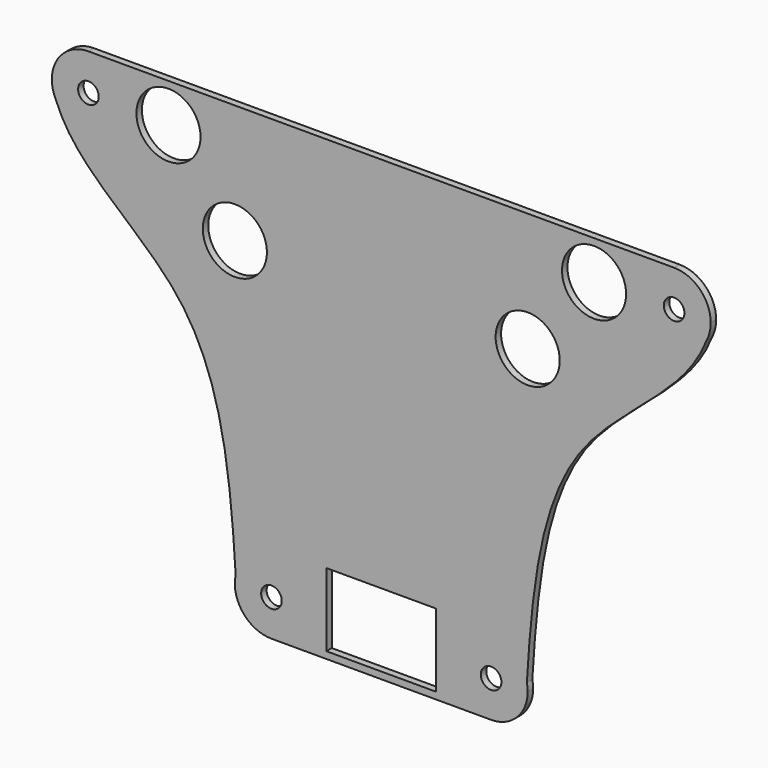
from build123d import *

# Parameters (mm, degrees)
F0_R     = 7.1501
F0_R_2   = 22.2504
F1_DEPTH = 4.7498


with BuildPart() as f1:
    # F0 (on Front) → F1 (new body)
    with BuildSketch(Plane.XZ):
        with BuildLine():
            ThreePointArc((-225.6573369788, 94.4161567678), (-197.0867504248, 81.6298943923), (-177.8, 106.2832548048))
            ThreePointArc((-177.8, 106.2832548048), (-185.2394877579, 124.2437670469), (-203.2, 131.6832548048))
            ThreePointArc((-203.2, 131.6832548048), (-224.9552785565, 119.3930929018), (-225.6573369788, 94.4161567678))
        make_face()
        with Locations((-203.2, 106.2832548048)):
            Circle(F0_R, mode=Mode.SUBTRACT)
        with BuildLine():
            ThreePointArc((-203.2, 131.6832548048), (-185.2394877579, 124.2437670469), (-177.8, 106.2832548048))
            ThreePointArc((-177.8, 106.2832548048), (-197.0867504248, 81.6298943923), (-225.6573369788, 94.4161567678))
            add(Edge.make_bspline(
                [(-225.6573369788, 94.4161567678), (-210.8833649868, 55.9874046479), (-115.4710726931, 10.7964254469), (-104.8309285082, -94.2151341667), (-101.0213270695, -155.0258526432)],
                knots=[0, 0, 0, 0, 0.4720003547, 1, 1, 1, 1], degree=3))
            ThreePointArc((-101.0213270695, -155.0258526432), (-73.4890691235, -135.1618277773), (-50.8, -160.4167451952))
            ThreePointArc((-50.8, -160.4167451952), (-58.2394877579, -178.3772574373), (-76.2, -185.8167451952))
            Line((-76.2, -185.8167451952), (76.2, -185.8167451952))
            ThreePointArc((76.2, -185.8167451952), (56.4251590294, -144.4757394368), (101.0213270695, -155.0258526432))
            add(Edge.make_bspline(
                [(225.6573369788, 94.4161567678), (210.8833649868, 55.9874046479), (115.4710726931, 10.7964254469), (104.8309285082, -94.2151341667), (101.0213270695, -155.0258526432)],
                knots=[0, 0, 0, 0, 0.4720003547, 1, 1, 1, 1], degree=3))
            ThreePointArc((225.6573369788, 94.4161567678), (181.4447214435, 93.1734167078), (203.2, 131.6832548048))
            Line((203.2, 131.6832548048), (-203.2, 131.6832548048))
        make_face()
        Polygon((-38.1, -130.2669451952), (0, -130.2669451952), (38.1, -130.2669451952), (38.1, -181.0669451952), (0, -181.0669451952), (-38.1, -181.0669451952), align=None, mode=Mode.SUBTRACT)
        with Locations((-101.6, 49.1332548048)):
            Circle(F0_R_2, mode=Mode.SUBTRACT)
        with Locations((-147.6502, 104.6830548048)):
            Circle(F0_R_2, mode=Mode.SUBTRACT)
        with Locations((101.6, 49.1332548048)):
            Circle(F0_R_2, mode=Mode.SUBTRACT)
        with Locations((147.6502, 104.6830548048)):
            Circle(F0_R_2, mode=Mode.SUBTRACT)
        with BuildLine():
            ThreePointArc((228.6, 106.2832548048), (221.1605122421, 124.2437670469), (203.2, 131.6832548048))
            ThreePointArc((203.2, 131.6832548048), (181.4447214435, 93.1734167078), (225.6573369788, 94.4161567678))
            ThreePointArc((225.6573369788, 94.4161567678), (227.8533604125, 100.1700052296), (228.6, 106.2832548048))
        make_face()
        with Locations((203.2, 106.2832548048)):
            Circle(F0_R, mode=Mode.SUBTRACT)
        with BuildLine():
            ThreePointArc((-50.8, -160.4167451952), (-73.4890691235, -135.1618277773), (-101.0213270695, -155.0258526432))
            ThreePointArc((-101.0213270695, -155.0258526432), (-95.9748409706, -176.3577509536), (-76.2, -185.8167451952))
            ThreePointArc((-76.2, -185.8167451952), (-58.2394877579, -178.3772574373), (-50.8, -160.4167451952))
        make_face()
        with Locations((-76.2, -160.4167451952)):
            Circle(F0_R, mode=Mode.SUBTRACT)
        with BuildLine():
            ThreePointArc((101.6, -160.4167451952), (101.4549174179, -157.7058143187), (101.0213270695, -155.0258526432))
            ThreePointArc((101.0213270695, -155.0258526432), (56.4251590294, -144.4757394368), (76.2, -185.8167451952))
            ThreePointArc((76.2, -185.8167451952), (94.1605122421, -178.3772574373), (101.6, -160.4167451952))
        make_face()
        with Locations((76.2, -160.4167451952)):
            Circle(F0_R, mode=Mode.SUBTRACT)
    extrude(amount=F1_DEPTH)


solid = f1.part
